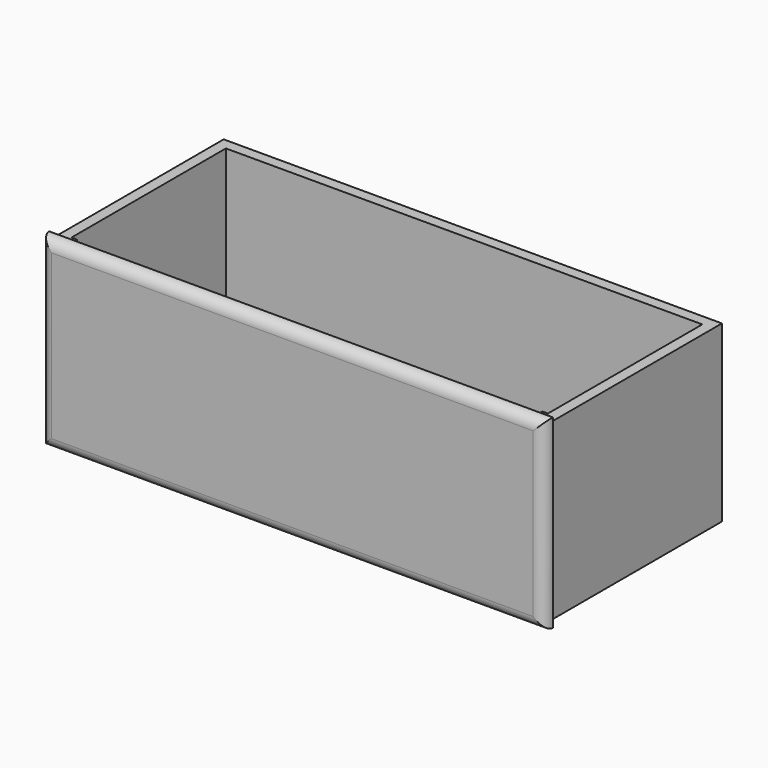
from build123d import *

# Parameters (mm, degrees)
F0_W     = 580.39
F0_H     = 250.19
F1_DEPTH = 101.6
F2_T     = -12.7
F3_W     = 542.29
F3_H     = 184.15
F4_DEPTH = 25.4
F5_W     = 586.74
F5_H     = 215.9
F6_DEPTH = 12.7
F7_R     = 12.69999


# Not quite as in the source:
# - a fillet or chamfer is up to 0.001 mm smaller than in the source, because OpenCascade refuses the exact size


with BuildPart() as f1:
    # F0 (on Top) → F1 (new body, symmetric)
    with BuildSketch(Plane.XY):
        Rectangle(F0_W, F0_H)
    extrude(amount=F1_DEPTH, both=True)

    # F2
    f2_openings = [f1.faces().sort_by_distance(p)[0] for p in [
        (0, 0, 101.6),
    ]]
    offset(amount=F2_T, openings=f2_openings)

    # F3 (on face) → F4 (cut)
    with BuildSketch(Plane.XZ.offset(125.095)):
        with Locations((0, 9.525)):
            Rectangle(F3_W, F3_H)
    extrude(amount=-F4_DEPTH, mode=Mode.SUBTRACT)

    # F5 (on face) → F6 (join)
    with BuildSketch(Plane.XZ.offset(125.095)):
        Rectangle(F5_W, F5_H)
        Polygon((-290.195, -101.6), (-290.195, 101.6), (-271.145, 101.6), (-271.145, -82.55), (271.145, -82.55), (271.145, 101.6), (290.195, 101.6), (290.195, -101.6), align=None, mode=Mode.SUBTRACT)
        Polygon((-271.145, 101.6), (-290.195, 101.6), (-290.195, -101.6), (290.195, -101.6), (290.195, 101.6), (271.145, 101.6), (271.145, -82.55), (-271.145, -82.55), align=None)
    extrude(amount=F6_DEPTH)

    # F7 (radius 12.7 in the source; OpenCascade refuses exactly that, so slightly less here)
    f7_edges = [f1.edges().sort_by_distance(p)[0] for p in [
        (0, -137.795, 107.95),
        (-293.37, -137.795, 0),
        (0, -137.795, -107.95),
        (293.37, -137.795, 0),
    ]]
    fillet(f7_edges, radius=F7_R)


solid = f1.part
